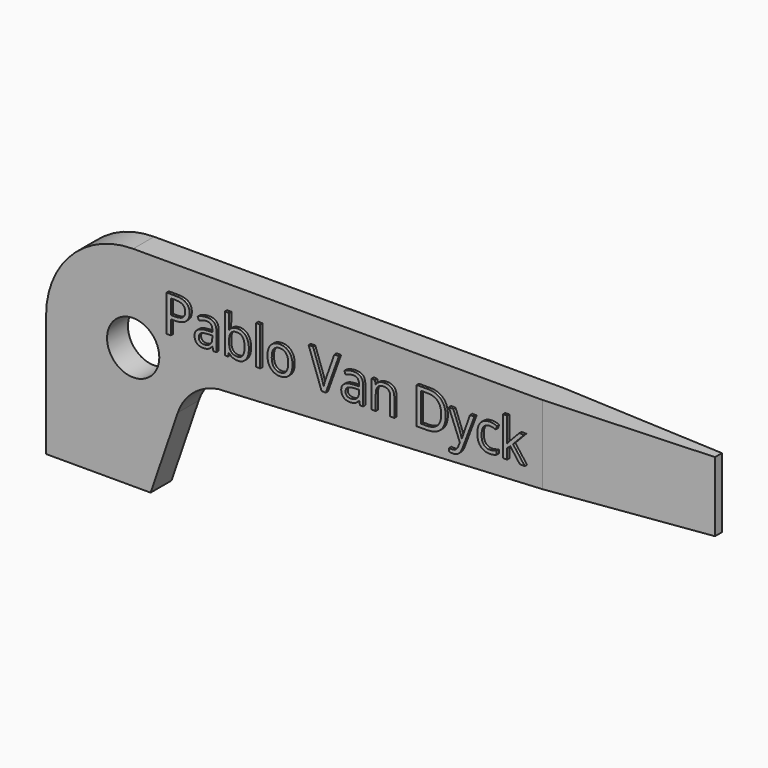
from build123d import *

# Parameters (mm, degrees)
F1_DEPTH     = 2.38125
F2_R         = 2.38125
F3_DEPTH     = 25.4
F5_DEPTH     = 25.4
F6_TEXT_SIZE = 4.6402123942
F7_DEPTH     = 0.254


# Not quite as in the source:
# - Text() gives the source's letters only with a copy of the font that has no kerning and outlines rounded to 1/6400 em; it was checked with that copy


with BuildPart() as f1:
    # F0 (on Front) → F1 (new body)
    with BuildSketch(Plane.XZ):
        with BuildLine():
            Line((60.325, 19.05), (7.9375, 19.05))
            ThreePointArc((7.9375, 19.05), (2.3248399243, 16.7251600757), (0, 11.1125))
            Line((0, 11.1125), (0, 0))
            Line((0, 0), (9.525, 0))
            Line((9.525, 0), (12.0040159672, 7.2256256826))
            ThreePointArc((12.0040159672, 7.2256256826), (13.4068357971, 9.2751561207), (15.6631963617, 10.3130942181))
            Line((15.6631963617, 10.3130942181), (60.325, 12.7))
            Line((60.325, 12.7), (60.325, 19.05))
        make_face()
    extrude(amount=F1_DEPTH)

    # F2 (on face) → F3 (cut)
    with BuildSketch(Plane.XZ.offset(2.38125)):
        with Locations((7.9375, 11.1125)):
            Circle(F2_R)
    extrude(amount=-F3_DEPTH, mode=Mode.SUBTRACT)

    # F4 (on face) → F5 (cut)
    with BuildSketch(Plane.XY.offset(19.05)):
        Polygon((60.325, -2.38125), (60.325, -1.5875), (45.24375, -2.38125), align=None)
        Polygon((45.24375, 0), (60.325, -0.79375), (60.325, 0), align=None)
    extrude(amount=-F5_DEPTH, mode=Mode.SUBTRACT)

    # F6 (on face) → F7 (join)
    with BuildSketch(Plane.XZ.offset(2.38125)):
        with Locations((10.7272670787, 13.3842071518)):
            Text('Pablo Van Dyck', F6_TEXT_SIZE, font='Open Sans', text_align=(TextAlign.LEFT, TextAlign.BOTTOM))
    extrude(amount=F7_DEPTH)


solid = f1.part
